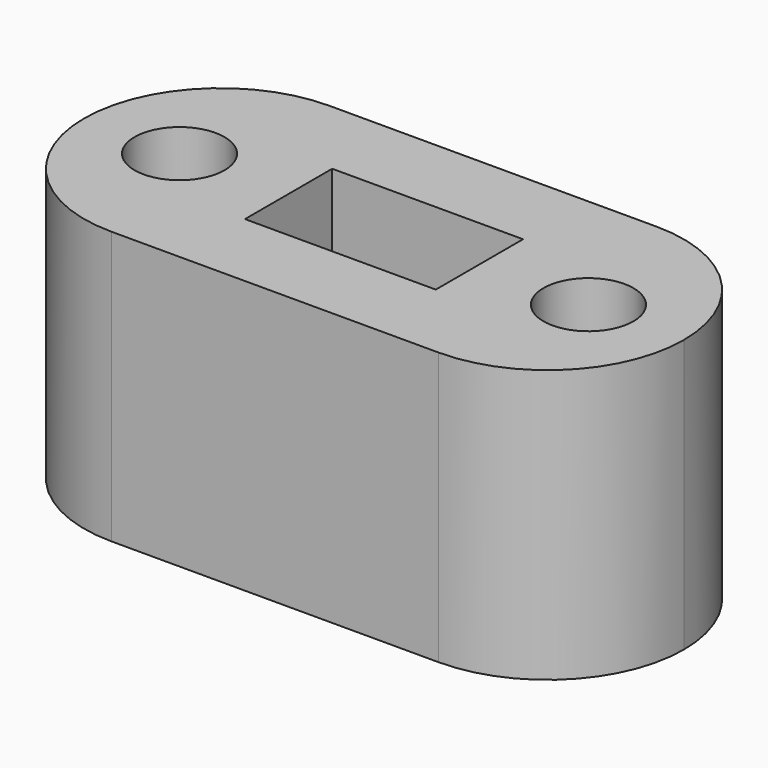
from build123d import *

# Parameters (mm, degrees)
F0_W     = 22
F0_H     = 10
F1_DEPTH = 10
F2_R     = 1.65
F2_W     = 7
F2_H     = 4
F3_DEPTH = 10.001
F4_R     = 4.99999


# Not quite as in the source:
# - a fillet or chamfer is up to 0.001 mm smaller than in the source, because OpenCascade refuses the exact size


with BuildPart() as f1:
    # F0 (on Top) → F1 (new body)
    with BuildSketch(Plane.XY):
        Rectangle(F0_W, F0_H)
    extrude(amount=F1_DEPTH)

    # F2 (on face) → F3 (cut, through all)
    with BuildSketch(Plane.XY.offset(10)):
        with Locations((-7.5, 0)):
            Circle(F2_R)
        with Locations((7.5, 0)):
            Circle(F2_R)
        Rectangle(F2_W, F2_H)
    extrude(amount=-F3_DEPTH, mode=Mode.SUBTRACT)

    # F4 (radius 5 in the source; OpenCascade refuses exactly that, so slightly less here)
    f4_edges = [f1.edges().sort_by_distance(p)[0] for p in [
        (-11, 5, 5),
        (-11, -5, 5),
        (11, 5, 5),
        (11, -5, 5),
    ]]
    fillet(f4_edges, radius=F4_R)


solid = f1.part
